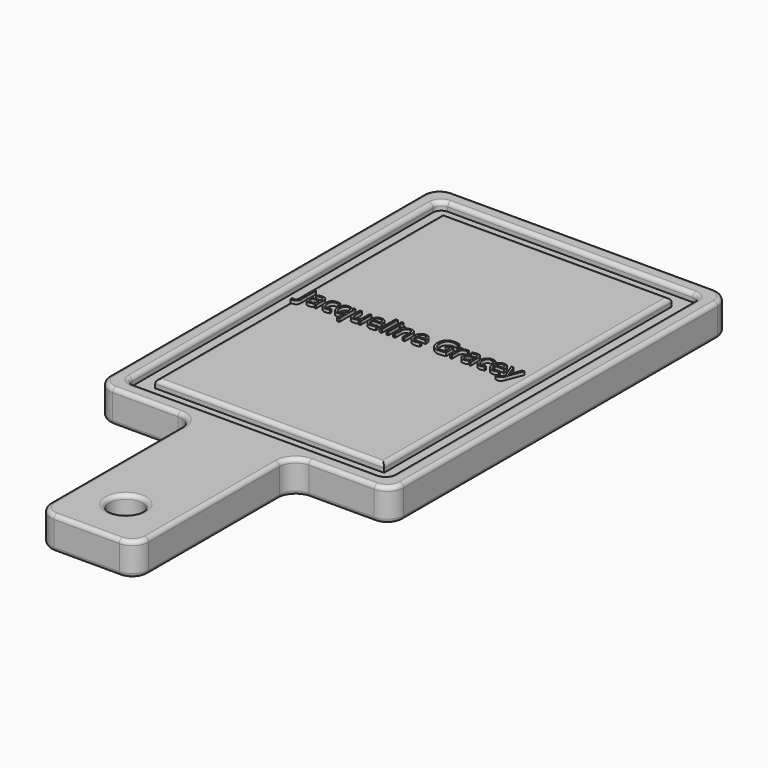
from build123d import *

# Parameters (mm, degrees)
F0_W         = 76.2
F0_H         = 152.4
F1_DEPTH     = 25.4
F2_R         = 12.7
F3_DEPTH     = 25.4
F5_DEPTH     = 6.35
F6_R         = 6.35
F7_R         = 12.7
F8_R         = 3.175
F9_TEXT_SIZE = 20.4035041228
F10_DEPTH    = 2.54


# Not quite as in the source:
# - Text() gives the source's letters only with a copy of the font that has no kerning and outlines rounded to 1/6400 em; it was checked with that copy


with BuildPart() as f1:
    # F0 (on Top) → F1 (new body)
    with BuildSketch(Plane.XY):
        Polygon((0, 330.2), (0, 0), (76.2, 0), (152.4, 0), (228.6, 0), (228.6, 330.2), align=None)
        with Locations((114.3, -76.2)):
            Rectangle(F0_W, F0_H)
    extrude(amount=F1_DEPTH)

    # F2 (on face) → F3 (cut)
    with BuildSketch(Plane.XY.offset(25.4)):
        with Locations((114.3, -114.3)):
            Circle(F2_R)
    extrude(amount=-F3_DEPTH, mode=Mode.SUBTRACT)

    # F4 (on face) → F5 (cut)
    with BuildSketch(Plane.XY.offset(25.4)):
        Polygon((12.7000047684, 12.7000047684), (76.2, 12.7000047684), (215.8999952316, 12.7000047684), (215.8999952316, 317.4999952316), (12.7000047684, 317.4999952316), align=None)
        Polygon((203.200003767, 304.800003767), (203.200003767, 25.399996233), (76.2, 25.399996233), (25.399996233, 25.399996233), (25.399996233, 304.800003767), align=None, mode=Mode.SUBTRACT)
    extrude(amount=-F5_DEPTH, mode=Mode.SUBTRACT)

    # F6
    f6_edges = [f1.edges().sort_by_distance(p)[0] for p in [
        (12.700005, 12.700005, 22.225),
        (215.899995, 12.700005, 22.225),
        (215.899995, 317.499995, 22.225),
        (12.700005, 317.499995, 22.225),
    ]]
    fillet(f6_edges, radius=F6_R)

    # F7
    f7_edges = [f1.edges().sort_by_distance(p)[0] for p in [
        (228.6, 0, 12.7),
        (152.4, -152.4, 12.7),
        (76.2, -152.4, 12.7),
        (228.6, 330.2, 12.7),
        (0, 0, 12.7),
        (0, 330.2, 12.7),
        (152.4, 0, 12.7),
        (76.2, 0, 12.7),
    ]]
    fillet(f7_edges, radius=F7_R)

    # F8
    f8_edges = [f1.edges().sort_by_distance(p)[0] for p in [
        (203.200004, 165.1, 25.4),
        (114.3, 25.399996, 25.4),
        (25.399996, 165.1, 25.4),
        (114.3, 304.800004, 25.4),
        (0, 165.1, 25.4),
        (3.719744, 326.480256, 25.4),
        (3.719744, 3.719744, 25.4),
        (114.3, 330.2, 25.4),
        (38.1, 0, 25.4),
        (224.880256, 326.480256, 25.4),
        (72.480256, -3.719744, 25.4),
        (228.6, 165.1, 25.4),
        (76.2, -76.2, 25.4),
        (224.880256, 3.719744, 25.4),
        (79.919744, -148.680256, 25.4),
        (190.5, 0, 25.4),
        (114.3, -152.4, 25.4),
        (156.119744, -3.719744, 25.4),
        (148.680256, -148.680256, 25.4),
        (152.4, -76.2, 25.4),
        (215.899995, 165.1, 25.4),
        (214.040123, 14.559877, 25.4),
        (214.040123, 315.640123, 25.4),
        (114.3, 12.700005, 25.4),
        (114.3, 317.499995, 25.4),
        (14.559877, 14.559877, 25.4),
        (14.559877, 315.640123, 25.4),
        (12.700005, 165.1, 25.4),
        (101.6, -114.3, 25.4),
        (0, 165.1, 0),
        (3.719744, 326.480256, 0),
        (3.719744, 3.719744, 0),
        (114.3, 330.2, 0),
        (38.1, 0, 0),
        (224.880256, 326.480256, 0),
        (72.480256, -3.719744, 0),
        (228.6, 165.1, 0),
        (76.2, -76.2, 0),
        (224.880256, 3.719744, 0),
        (79.919744, -148.680256, 0),
        (190.5, 0, 0),
        (114.3, -152.4, 0),
        (156.119744, -3.719744, 0),
        (148.680256, -148.680256, 0),
        (152.4, -76.2, 0),
        (101.6, -114.3, 0),
    ]]
    fillet(f8_edges, radius=F8_R)

    # F9 (on face) → F10 (join)
    with BuildSketch(Plane.XY.offset(25.4)):
        with Locations((28.574996233, 158.6046153904)):
            Text('Jacqueline Gracey', F9_TEXT_SIZE, font='Open Sans', text_align=(TextAlign.LEFT, TextAlign.BOTTOM))
    extrude(amount=F10_DEPTH)


solid = f1.part
